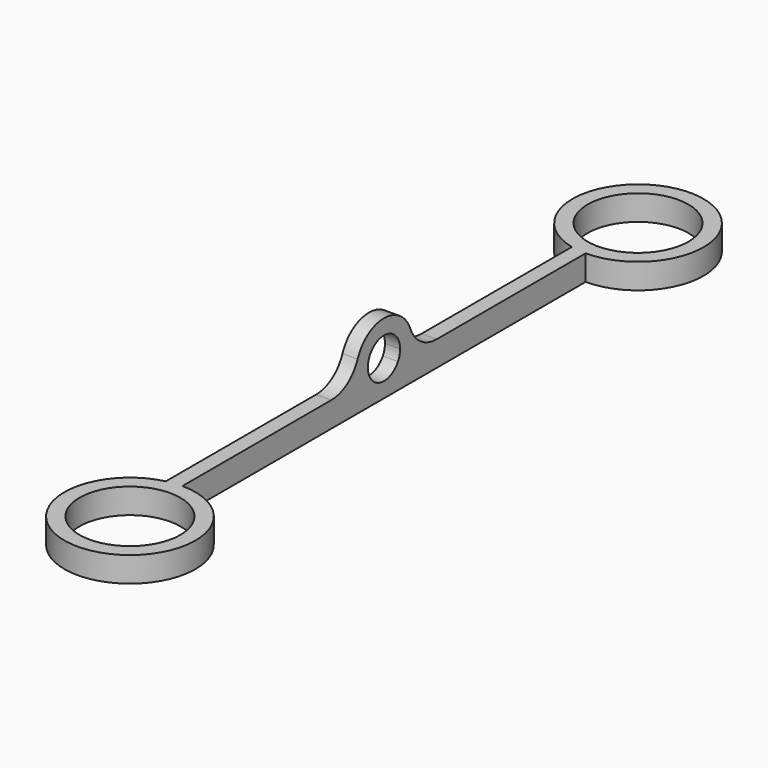
from build123d import *
from build123d import SkipClean  # not in build123d's __all__

# Parameters (mm, degrees)
F0_R     = 10
F1_DEPTH = 2.5
F3_DEPTH = 3
F4_DEPTH = 25


# Not quite as in the source:
# - a feature names something its author has since deleted; it is built from what else it names


with BuildPart() as f1:
    # F0 (on Top) → F1 (new body, symmetric)
    with BuildSketch(Plane.XY):
        with BuildLine():
            Line((-3, 50.3508893593), (-3, -50.3508893593))
            ThreePointArc((-3, -50.3508893593), (1.5102254254, -75.9119796764), (0, -50))
            Line((0, -50), (0, 50))
            ThreePointArc((0, 50), (1.5102254254, 75.9119796764), (-3, 50.3508893593))
        make_face()
        with Locations((0, -63)):
            Circle(F0_R, mode=Mode.SUBTRACT)
        with Locations((0, 63)):
            Circle(F0_R, mode=Mode.SUBTRACT)
    extrude(amount=F1_DEPTH, both=True)

    # F2 (on face) → F3 (join, through all)
    with BuildSketch(Plane.YZ):
        with BuildLine():
            ThreePointArc((-3.4641016151, 2.5), (-1.0352761804, 8.3637033052), (4, 4.5))
            ThreePointArc((4, 4.5), (3.8637033052, 3.4647238196), (3.4641016151, 2.5))
            Line((3.4641016151, 2.5), (13.0766968306, 2.5))
            ThreePointArc((13.0766968306, 2.5), (9.108069864, 3.7337187027), (6.5383484153, 7))
            ThreePointArc((6.5383484153, 7), (0, 11.5), (-6.5383484153, 7))
            ThreePointArc((-6.5383484153, 7), (-9.108069864, 3.7337187027), (-13.0766968306, 2.5))
            Line((-13.0766968306, 2.5), (-3.4641016151, 2.5))
        make_face()
        with BuildLine():
            ThreePointArc((3.4641016151, 2.5), (0, 0.5), (-3.4641016151, 2.5))
            Line((-3.4641016151, 2.5), (-13.0766968306, 2.5))
            Line((-13.0766968306, 2.5), (-13.0766968306, -2.5))
            Line((-13.0766968306, -2.5), (13.0766968306, -2.5))
            Line((13.0766968306, -2.5), (13.0766968306, 2.5))
            Line((13.0766968306, 2.5), (3.4641016151, 2.5))
        make_face()
    extrude(amount=-F3_DEPTH)

    # F2 (on face) → F4 (cut)
    with BuildSketch(Plane.YZ):
        with BuildLine():
            Line((3.4641016151, 2.5), (-3.4641016151, 2.5))
            ThreePointArc((-3.4641016151, 2.5), (0, 0.5), (3.4641016151, 2.5))
        make_face()
    with SkipClean():  # cleaning this boolean's faces spoils the solid; the shape is the same uncleaned
        extrude(amount=-F4_DEPTH, mode=Mode.SUBTRACT)


solid = f1.part
